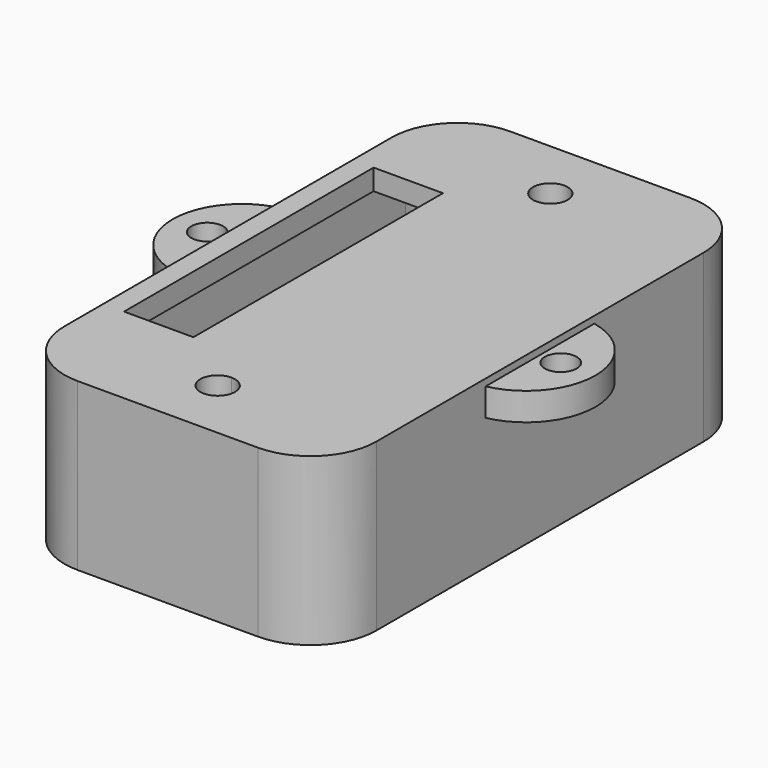
from build123d import *

# Parameters (mm, degrees)
F0_R     = 2.5
F1_DEPTH = 2
F2_DEPTH = 23
F3_DEPTH = 3
F0_R_2   = 2.297943
F4_DEPTH = 2
F5_DEPTH = 1
F6_DEPTH = 2


# Not quite as in the source:
# - a feature names something its author has since deleted; it is built from what else it names


with BuildPart() as f1:
    # F0 (on Top) → F1 (new body)
    with BuildSketch(Plane.XY):
        with BuildLine():
            Line((-13, -37), (13, -37))
            ThreePointArc((13, -37), (18.303301, -34.803301), (20.5, -29.5))
            Line((20.5, -29.5), (20.5, 29.5))
            ThreePointArc((20.5, 29.5), (18.303301, 34.803301), (13, 37))
            Line((13, 37), (-13, 37))
            ThreePointArc((-13, 37), (-18.303301, 34.803301), (-20.5, 29.5))
            Line((-20.5, 29.5), (-20.5, -29.5))
            ThreePointArc((-20.5, -29.5), (-18.303301, -34.803301), (-13, -37))
        make_face()
        with BuildLine():
            ThreePointArc((0, -27.5), (1.767767, -28.232233), (2.5, -30))
            ThreePointArc((2.5, -30), (-1.767767, -31.767767), (0, -27.5))
        make_face(mode=Mode.SUBTRACT)
        Polygon((-19.5, -22.5), (-19.5, 0), (-19.5, 22.5), (-9.5, 22.5), (-9.5, 0), (-9.5, -22.5), align=None, mode=Mode.SUBTRACT)
        with Locations((0, 30)):
            Circle(F0_R, mode=Mode.SUBTRACT)
    extrude(amount=-F1_DEPTH)

    # F0 (on Top) → F2 (join)
    with BuildSketch(Plane.XY):
        with BuildLine():
            Line((-22.5, -9.797959), (-22.5, -29.5))
            ThreePointArc((-22.5, -29.5), (-19.717514, -36.217514), (-13, -39))
            Line((-13, -39), (13, -39))
            ThreePointArc((13, -39), (19.717514, -36.217514), (22.5, -29.5))
            Line((22.5, -29.5), (22.5, -9.797959))
            Line((22.5, -9.797959), (22.5, 0))
            Line((22.5, 0), (22.5, 9.797959))
            Line((22.5, 9.797959), (22.5, 29.5))
            ThreePointArc((22.5, 29.5), (19.717514, 36.217514), (13, 39))
            Line((13, 39), (-13, 39))
            ThreePointArc((-13, 39), (-19.717514, 36.217514), (-22.5, 29.5))
            Line((-22.5, 29.5), (-22.5, 9.797959))
            Line((-22.5, 9.797959), (-22.5, -9.797959))
        make_face()
        with BuildLine():
            ThreePointArc((20.5, -29.5), (18.303301, -34.803301), (13, -37))
            Line((13, -37), (-13, -37))
            ThreePointArc((-13, -37), (-18.303301, -34.803301), (-20.5, -29.5))
            Line((-20.5, -29.5), (-20.5, 29.5))
            ThreePointArc((-20.5, 29.5), (-18.303301, 34.803301), (-13, 37))
            Line((-13, 37), (13, 37))
            ThreePointArc((13, 37), (18.303301, 34.803301), (20.5, 29.5))
            Line((20.5, 29.5), (20.5, -29.5))
        make_face(mode=Mode.SUBTRACT)
    extrude(amount=-F2_DEPTH)

    # F3 (add): a face of the model
    f3_faces = [f1.faces().sort_by_distance(p)[0] for p in [
        (2.613717, 0, -2),
    ]]
    extrude(f3_faces, amount=-F3_DEPTH)

    # F0 (on Top) → F4 (join)
    with BuildSketch(Plane.XY):
        with BuildLine():
            Line((-22.5, -9.797959), (-22.5, -29.5))
            ThreePointArc((-22.5, -29.5), (-19.717514, -36.217514), (-13, -39))
            Line((-13, -39), (13, -39))
            ThreePointArc((13, -39), (19.717514, -36.217514), (22.5, -29.5))
            Line((22.5, -29.5), (22.5, -9.797959))
            Line((22.5, -9.797959), (22.5, 0))
            Line((22.5, 0), (22.5, 9.797959))
            Line((22.5, 9.797959), (22.5, 29.5))
            ThreePointArc((22.5, 29.5), (19.717514, 36.217514), (13, 39))
            Line((13, 39), (-13, 39))
            ThreePointArc((-13, 39), (-19.717514, 36.217514), (-22.5, 29.5))
            Line((-22.5, 29.5), (-22.5, 9.797959))
            Line((-22.5, 9.797959), (-22.5, -9.797959))
        make_face()
        with BuildLine():
            ThreePointArc((20.5, -29.5), (18.303301, -34.803301), (13, -37))
            Line((13, -37), (-13, -37))
            ThreePointArc((-13, -37), (-18.303301, -34.803301), (-20.5, -29.5))
            Line((-20.5, -29.5), (-20.5, 29.5))
            ThreePointArc((-20.5, 29.5), (-18.303301, 34.803301), (-13, 37))
            Line((-13, 37), (13, 37))
            ThreePointArc((13, 37), (18.303301, 34.803301), (20.5, 29.5))
            Line((20.5, 29.5), (20.5, -29.5))
        make_face(mode=Mode.SUBTRACT)
        with BuildLine():
            ThreePointArc((-22.5, 9.797959), (-30.5, 0), (-22.5, -9.797959))
            Line((-22.5, -9.797959), (-22.5, 9.797959))
        make_face()
        with Locations((-25.5, 0)):
            Circle(F0_R_2, mode=Mode.SUBTRACT)
        with BuildLine():
            Line((22.5, 0), (22.5, -9.797959))
            ThreePointArc((22.5, -9.797959), (30.5, 0), (22.5, 9.797959))
            Line((22.5, 9.797959), (22.5, 0))
        make_face()
        with BuildLine():
            ThreePointArc((27.797943, 0), (25.5, -2.297943), (23.202057, 0))
            ThreePointArc((23.202057, 0), (25.5, 2.297943), (27.797943, 0))
        make_face(mode=Mode.SUBTRACT)
    extrude(amount=-F4_DEPTH)

    # F0 (on Top) → F5 (join)
    with BuildSketch(Plane.XY):
        with BuildLine():
            Line((-22.5, -9.797959), (-22.5, -29.5))
            ThreePointArc((-22.5, -29.5), (-19.717514, -36.217514), (-13, -39))
            Line((-13, -39), (13, -39))
            ThreePointArc((13, -39), (19.717514, -36.217514), (22.5, -29.5))
            Line((22.5, -29.5), (22.5, -9.797959))
            Line((22.5, -9.797959), (22.5, 0))
            Line((22.5, 0), (22.5, 9.797959))
            Line((22.5, 9.797959), (22.5, 29.5))
            ThreePointArc((22.5, 29.5), (19.717514, 36.217514), (13, 39))
            Line((13, 39), (-13, 39))
            ThreePointArc((-13, 39), (-19.717514, 36.217514), (-22.5, 29.5))
            Line((-22.5, 29.5), (-22.5, 9.797959))
            Line((-22.5, 9.797959), (-22.5, -9.797959))
        make_face()
        with BuildLine():
            ThreePointArc((20.5, -29.5), (18.303301, -34.803301), (13, -37))
            Line((13, -37), (-13, -37))
            ThreePointArc((-13, -37), (-18.303301, -34.803301), (-20.5, -29.5))
            Line((-20.5, -29.5), (-20.5, 29.5))
            ThreePointArc((-20.5, 29.5), (-18.303301, 34.803301), (-13, 37))
            Line((-13, 37), (13, 37))
            ThreePointArc((13, 37), (18.303301, 34.803301), (20.5, 29.5))
            Line((20.5, 29.5), (20.5, -29.5))
        make_face(mode=Mode.SUBTRACT)
    extrude(amount=F5_DEPTH)

    # F6 (add): faces of the model
    f6_faces = [f1.faces().sort_by_distance(p)[0] for p in [
        (-30.28834, 0, -2),
        (22.71166, 0, -2),
    ]]
    extrude(f6_faces, amount=F6_DEPTH)


solid = f1.part
